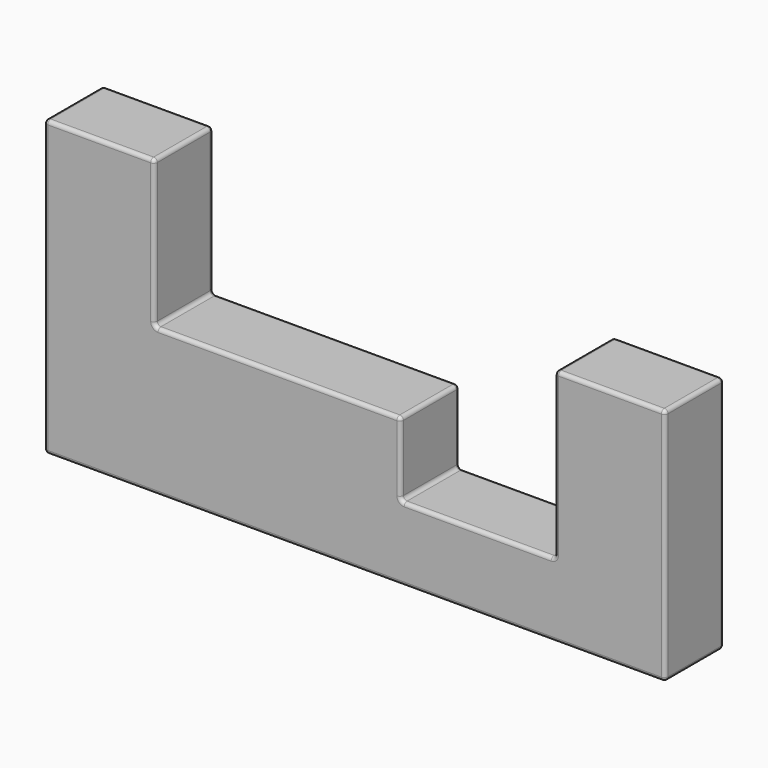
from build123d import *

# Parameters (mm, degrees)
F1_DEPTH     = 20
F2_F1_R      = 1
F2_F2_R      = 1
F3_T1_DEPTH  = 63
F3_T3_DEPTH  = 28
F3_T5_DEPTH  = 167
F3_T7_DEPTH  = 78
F3_S11_W     = 1
F3_S11_H     = 1
F3_T12_DEPTH = 1
F3_S17_W     = 1
F3_S17_H     = 1
F3_T18_DEPTH = 1
F3_T22_ANGLE = 90
F3_T24_ANGLE = 90
F3_T26_ANGLE = 90


# Not quite as in the source:
# - a fillet or chamfer that OpenCascade refuses, or shapes differently, is made with other operations: its cross-section is extruded or revolved along the edge and cut away or added


with BuildPart() as f1:
    # F0 (on Front) → F1 (new body)
    with BuildSketch(Plane.XZ):
        Polygon((-54.7987632453, 48.7000103295), (-54.7987632453, -31.2999896705), (114.2012367547, -31.2999896705), (114.2012367547, 33.7000103295), (84.2012367547, 33.7000103295), (84.2012367547, -11.2999896705), (42.2012367547, -11.2999896705), (42.2012367547, 8.7000103295), (-24.7987632453, 8.7000103295), (-24.7987632453, 48.7000103295), align=None)
    extrude(amount=F1_DEPTH)

    # F2: fillet of radius 1 on 24 edges, made by hand

    # F2_f1
    f2_f1_edges = [f1.edges().sort_by_distance(p)[0] for p in [
        (-24.7987632453, -10, 8.7000103295),
        (84.2012367547, -10, -11.2999896705),
        (42.2012367547, -10, -11.2999896705),
    ]]
    fillet(f2_f1_edges, radius=F2_F1_R)

    # F2_f2
    f2_f2_edges = [f1.edges().sort_by_distance(p)[0] for p in [
        (-39.7987632453, -20, 48.7000103295),
        (9.2012367547, -20, 8.7000103295),
        (-24.7987632453, -20, 29.2000103295),
        (9.2012367547, 0, 8.7000103295),
        (-24.7987632453, -10, 48.7000103295),
        (42.2012367547, -10, 8.7000103295),
        (42.2012367547, -20, -0.7999896705),
        (63.2012367547, 0, -11.2999896705),
        (63.2012367547, -20, -11.2999896705),
        (114.2012367547, -10, 33.7000103295),
        (114.2012367547, 0, 1.2000103295),
        (99.2012367547, 0, 33.7000103295),
        (84.2012367547, 0, 11.7000103295),
        (-54.7987632453, 0, 8.7000103295),
        (29.7012367547, 0, -31.2999896705),
        (-54.7987632453, -10, -31.2999896705),
        (84.2012367547, -10, 33.7000103295),
        (-24.7987632453, 0, 29.2000103295),
        (-39.7987632453, 0, 48.7000103295),
        (114.2012367547, -10, -31.2999896705),
        (-54.7987632453, -10, 48.7000103295),
        (-24.5058700265, 0, 8.9929035483),
        (83.9083435358, 0, -11.0070964517),
        (83.9083435358, -20, -11.0070964517),
        (42.4941299735, -20, -11.0070964517),
        (42.4941299735, 0, -11.0070964517),
        (-24.5058700265, -20, 8.9929035483),
    ]]
    fillet(f2_f2_edges, radius=F2_F2_R)

    # F3: fillet of radius 1 on 7 edges, made by hand

    # F3_s2 → F3_t1 (cut)
    with BuildSketch(Plane.XY.offset(-30.2999896705)):
        with BuildLine():
            ThreePointArc((113.2012367547, -20), (113.9083435358, -19.7071067812), (114.2012367547, -19))
            Line((114.2012367547, -19), (114.2012367547, -20))
            Line((114.2012367547, -20), (113.2012367547, -20))
        make_face()
    extrude(amount=F3_T1_DEPTH, mode=Mode.SUBTRACT)

    # F3_s4 → F3_t3 (cut)
    with BuildSketch(Plane.YZ.offset(85.2012367547)):
        with BuildLine():
            ThreePointArc((-20, 32.7000103295), (-19.7071067812, 33.4071171107), (-19, 33.7000103295))
            Line((-19, 33.7000103295), (-20, 33.7000103295))
            Line((-20, 33.7000103295), (-20, 32.7000103295))
        make_face()
    extrude(amount=F3_T3_DEPTH, mode=Mode.SUBTRACT)

    # F3_s6 → F3_t5 (cut)
    with BuildSketch(Plane.YZ.offset(-53.7987632453)):
        with BuildLine():
            ThreePointArc((-20, -30.2999896705), (-19.7071067812, -31.0070964517), (-19, -31.2999896705))
            Line((-19, -31.2999896705), (-20, -31.2999896705))
            Line((-20, -31.2999896705), (-20, -30.2999896705))
        make_face()
    extrude(amount=F3_T5_DEPTH, mode=Mode.SUBTRACT)

    # F3_s8 → F3_t7 (cut)
    with BuildSketch(Plane.XY.offset(-30.2999896705)):
        with BuildLine():
            ThreePointArc((-53.7987632453, -20), (-54.5058700265, -19.7071067812), (-54.7987632453, -19))
            Line((-54.7987632453, -19), (-54.7987632453, -20))
            Line((-54.7987632453, -20), (-53.7987632453, -20))
        make_face()
    extrude(amount=F3_T7_DEPTH, mode=Mode.SUBTRACT)


with BuildPart() as f3_tool10:
    # F3_s11 → F3_t12 (new body)
    with BuildSketch(Plane.XZ.offset(19)):
        with Locations((-54.2987632453, 48.2000103295)):
            Rectangle(F3_S11_W, F3_S11_H)
    extrude(amount=F3_T12_DEPTH)

    # F3_s13 → F3_t14 (revolve, cut)
    with BuildSketch(Plane(origin=(-53.7987632453, -19, 47.7000103295), x_dir=(0.7071067812, 0, -0.7071067812), z_dir=(-0.7071067812, 0, -0.7071067812))):
        with BuildLine():
            ThreePointArc((0, -1), (1, 0), (0, 1))
            Line((0, 1), (0, -1))
        make_face()
    revolve(axis=Axis((-53.7987632453, -19, 47.7000103295), (0, -1, 0)), mode=Mode.SUBTRACT)


with BuildPart() as f1_1:
    add(f1.part)

    # F3_t9: cut F3_tool10
    add(f3_tool10.part, mode=Mode.SUBTRACT)


with BuildPart() as f3_tool16:
    # F3_s17 → F3_t18 (new body)
    with BuildSketch(Plane.XZ.offset(19)):
        with Locations((84.7012367547, 33.2000103295)):
            Rectangle(F3_S17_W, F3_S17_H)
    extrude(amount=F3_T18_DEPTH)

    # F3_s19 → F3_t20 (revolve, cut)
    with BuildSketch(Plane(origin=(85.2012367547, -19, 32.7000103295), x_dir=(0.7071067812, 0, -0.7071067812), z_dir=(-0.7071067812, 0, -0.7071067812))):
        with BuildLine():
            ThreePointArc((0, -1), (1, 0), (0, 1))
            Line((0, 1), (0, -1))
        make_face()
    revolve(axis=Axis((85.2012367547, -19, 32.7000103295), (0, -1, 0)), mode=Mode.SUBTRACT)


with BuildPart() as f1_2:
    add(f1_1.part)

    # F3_t15: cut F3_tool16
    add(f3_tool16.part, mode=Mode.SUBTRACT)

    # F3_s21 → F3_t22 (revolve, cut)
    with BuildSketch(Plane.YZ.offset(113.2012367547)):
        with BuildLine():
            ThreePointArc((-20, 32.7000103295), (-19.7071067812, 33.4071171107), (-19, 33.7000103295))
            Line((-19, 33.7000103295), (-20, 33.7000103295))
            Line((-20, 33.7000103295), (-20, 32.7000103295))
        make_face()
    revolve(axis=Axis((113.2012367547, -20, 32.7000103295), (0, 1, 0)), revolution_arc=F3_T22_ANGLE, mode=Mode.SUBTRACT)

    # F3_s23 → F3_t24 (revolve, cut)
    with BuildSketch(Plane.XY.offset(-30.2999896705)):
        with BuildLine():
            ThreePointArc((113.2012367547, -20), (113.9083435358, -19.7071067812), (114.2012367547, -19))
            Line((114.2012367547, -19), (114.2012367547, -20))
            Line((114.2012367547, -20), (113.2012367547, -20))
        make_face()
    revolve(axis=Axis((113.2012367547, -20, -30.2999896705), (0, 1, 0)), revolution_arc=F3_T24_ANGLE, mode=Mode.SUBTRACT)

    # F3_s25 → F3_t26 (revolve, cut)
    with BuildSketch(Plane.YZ.offset(-53.7987632453)):
        with BuildLine():
            ThreePointArc((-20, -30.2999896705), (-19.7071067812, -31.0070964517), (-19, -31.2999896705))
            Line((-19, -31.2999896705), (-20, -31.2999896705))
            Line((-20, -31.2999896705), (-20, -30.2999896705))
        make_face()
    revolve(axis=Axis((-53.7987632453, -20, -30.2999896705), (0, 1, 0)), revolution_arc=F3_T26_ANGLE, mode=Mode.SUBTRACT)


solid = f1_2.part
